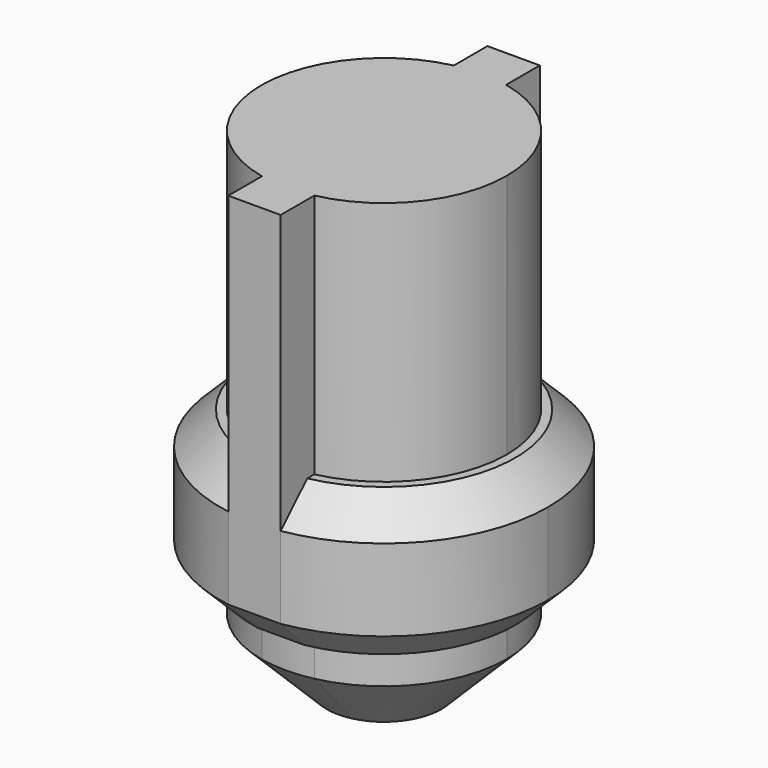
from build123d import *

# Parameters (mm, degrees)
F1_DEPTH     = 7.5
F2_DEPTH     = 7.5
F3_DEPTH     = 4.5
F4_SIZE      = 2
F5_T1_DEPTH  = 6.7433659759
F5_T4_ANGLE  = 220.4864882976
F5_T6_ANGLE  = 220.4864882976
F5_T10_ANGLE = 220.4864882976
F5_T15_ANGLE = 220.4864882976
F5_T20_ANGLE = 220.4864882976
F5_T25_ANGLE = 220.4864882976


# Not quite as in the source:
# - a fillet or chamfer that OpenCascade refuses, or shapes differently, is made with other operations: its cross-section is extruded or revolved along the edge and cut away or added


with BuildPart() as f1:
    # F0 (on Top) → F1 (new body)
    with BuildSketch(Plane.XY):
        with BuildLine():
            ThreePointArc((0.8, -3.6636730203), (2.9208303614, -2.3518609653), (3.75, 0))
            ThreePointArc((3.75, 0), (2.9208303614, 2.3518609653), (0.8, 3.6636730203))
            Line((0.8, 3.6636730203), (0.8, -3.6636730203))
        make_face()
        with BuildLine():
            Line((0.8, -3.6636730203), (0.8, 3.6636730203))
            ThreePointArc((0.8, 3.6636730203), (0, 3.75), (-0.8, 3.6636730203))
            Line((-0.8, 3.6636730203), (-0.8, -3.6636730203))
            ThreePointArc((-0.8, -3.6636730203), (0, -3.75), (0.8, -3.6636730203))
        make_face()
        with BuildLine():
            Line((-0.8, -3.6636730203), (-0.8, 3.6636730203))
            ThreePointArc((-0.8, 3.6636730203), (-3.75, 0), (-0.8, -3.6636730203))
        make_face()
    extrude(amount=-F1_DEPTH)

    # F0 (on Top) → F2 (join)
    with BuildSketch(Plane.XY):
        with BuildLine():
            ThreePointArc((0.8, -3.6636730203), (2.9208303614, -2.3518609653), (3.75, 0))
            ThreePointArc((3.75, 0), (2.9208303614, 2.3518609653), (0.8, 3.6636730203))
            Line((0.8, 3.6636730203), (0.8, -3.6636730203))
        make_face()
        with BuildLine():
            Line((0.8, -3.6636730203), (0.8, 3.6636730203))
            ThreePointArc((0.8, 3.6636730203), (0, 3.75), (-0.8, 3.6636730203))
            Line((-0.8, 3.6636730203), (-0.8, -3.6636730203))
            ThreePointArc((-0.8, -3.6636730203), (0, -3.75), (0.8, -3.6636730203))
        make_face()
        with BuildLine():
            Line((-0.8, -3.6636730203), (-0.8, 3.6636730203))
            ThreePointArc((-0.8, 3.6636730203), (-3.75, 0), (-0.8, -3.6636730203))
        make_face()
        with BuildLine():
            ThreePointArc((-0.8, 3.6636730203), (0, 3.75), (0.8, 3.6636730203))
            Line((0.8, 3.6636730203), (0.8, 4.95))
            Line((0.8, 4.95), (-0.8, 4.95))
            Line((-0.8, 4.95), (-0.8, 3.6636730203))
        make_face()
        with BuildLine():
            Line((0.8, -4.95), (0.8, -3.6636730203))
            ThreePointArc((0.8, -3.6636730203), (0, -3.75), (-0.8, -3.6636730203))
            Line((-0.8, -3.6636730203), (-0.8, -4.95))
            Line((-0.8, -4.95), (0.8, -4.95))
        make_face()
    extrude(amount=F2_DEPTH)

    # F0 (on Top) → F3 (join)
    with BuildSketch(Plane.XY):
        with BuildLine():
            ThreePointArc((0.8, 3.6636730203), (2.9208303614, 2.3518609653), (3.75, 0))
            ThreePointArc((3.75, 0), (2.9208303614, -2.3518609653), (0.8, -3.6636730203))
            Line((0.8, -3.6636730203), (0.8, -4.95))
            ThreePointArc((0.8, -4.95), (3.8179761524, -3.2504704428), (5.0142297514, 0))
            ThreePointArc((5.0142297514, 0), (3.8179761524, 3.2504704428), (0.8, 4.95))
            Line((0.8, 4.95), (0.8, 3.6636730203))
        make_face()
        with BuildLine():
            Line((0.8, -4.95), (0.8, -3.6636730203))
            ThreePointArc((0.8, -3.6636730203), (0, -3.75), (-0.8, -3.6636730203))
            Line((-0.8, -3.6636730203), (-0.8, -4.95))
            Line((-0.8, -4.95), (0.8, -4.95))
        make_face()
        with BuildLine():
            ThreePointArc((-0.8, -3.6636730203), (-3.75, 0), (-0.8, 3.6636730203))
            Line((-0.8, 3.6636730203), (-0.8, 4.95))
            ThreePointArc((-0.8, 4.95), (-5.0142297514, 0), (-0.8, -4.95))
            Line((-0.8, -4.95), (-0.8, -3.6636730203))
        make_face()
        with BuildLine():
            ThreePointArc((-0.8, 3.6636730203), (0, 3.75), (0.8, 3.6636730203))
            Line((0.8, 3.6636730203), (0.8, 4.95))
            Line((0.8, 4.95), (-0.8, 4.95))
            Line((-0.8, 4.95), (-0.8, 3.6636730203))
        make_face()
    extrude(amount=-F3_DEPTH)

    # F4
    f4_edges = [f1.edges().sort_by_distance(p)[0] for p in [
        (0.8, -3.663673, -7.5),
    ]]
    chamfer(f4_edges, length=F4_SIZE)

    # F5: chamfer of 1 on 6 edges, made by hand

    # F5_s2 → F5_t1 (cut)
    with BuildSketch(Plane.YZ.offset(-3.371682988)):
        Polygon((-3.95, -4.5), (-4.95, -3.5), (-4.95, -4.5), align=None)
        Polygon((3.95, -4.5), (4.95, -3.5), (4.95, -4.5), align=None)
    extrude(amount=F5_T1_DEPTH, mode=Mode.SUBTRACT)

    # F5_s3 → F5_t4 (revolve, cut)
    with BuildSketch(Plane(origin=(0, 0, 0), x_dir=(0, 0, 1), z_dir=(0.9382321407, -0.3460064308, 0))):
        Polygon((-4.5, -4.0142297514), (-3.5, -5.0142297514), (-4.5, -5.0142297514), align=None)
    revolve(axis=Axis((0, 0, -4.5), (0, 0, 1)), revolution_arc=F5_T4_ANGLE, mode=Mode.SUBTRACT)

    # F5_s5 → F5_t6 (revolve, cut)
    with BuildSketch(Plane(origin=(0, 0, 0), x_dir=(0, 0, 1), z_dir=(-0.9382321407, 0.3460064308, 0))):
        Polygon((-4.5, -4.0142297514), (-3.5, -5.0142297514), (-4.5, -5.0142297514), align=None)
    revolve(axis=Axis((0, 0, -4.5), (0, 0, 1)), revolution_arc=F5_T6_ANGLE, mode=Mode.SUBTRACT)


with BuildPart() as f5_tool8:
    # F5_s9 → F5_t10 (revolve)
    with BuildSketch(Plane(origin=(0, 0, 0), x_dir=(0, 0, 1), z_dir=(0.9382321407, -0.3460064308, 0))):
        Polygon((-1, -5.0142297514), (0, -4.0142297514), (0, -5.0142297514), align=None)
    revolve(axis=Axis((0, 0, 0), (0, 0, 1)), revolution_arc=F5_T10_ANGLE)

    split(bisect_by=Plane.YZ.offset(0.8), keep=Keep.TOP)


with BuildPart() as f1_1:
    add(f1.part)

    # F5_t7: cut F5_tool8
    add(f5_tool8.part, mode=Mode.SUBTRACT)


with BuildPart() as f5_tool13:
    # F5_s14 → F5_t15 (revolve)
    with BuildSketch(Plane(origin=(0, 0, 0), x_dir=(0, 0, 1), z_dir=(0.9382321407, -0.3460064308, 0))):
        Polygon((-1, -5.0142297514), (0, -4.0142297514), (0, -5.0142297514), align=None)
    revolve(axis=Axis((0, 0, 0), (0, 0, 1)), revolution_arc=F5_T15_ANGLE)

    split(bisect_by=Plane.YZ.offset(-0.8), keep=Keep.BOTTOM)


with BuildPart() as f1_2:
    add(f1_1.part)

    # F5_t12: cut F5_tool13
    add(f5_tool13.part, mode=Mode.SUBTRACT)


with BuildPart() as f5_tool18:
    # F5_s19 → F5_t20 (revolve)
    with BuildSketch(Plane(origin=(0, 0, 0), x_dir=(0, 0, 1), z_dir=(-0.9382321407, 0.3460064308, 0))):
        Polygon((-1, -5.0142297514), (0, -4.0142297514), (0, -5.0142297514), align=None)
    revolve(axis=Axis((0, 0, 0), (0, 0, 1)), revolution_arc=F5_T20_ANGLE)

    split(bisect_by=Plane.YZ.offset(-0.8), keep=Keep.BOTTOM)


with BuildPart() as f1_3:
    add(f1_2.part)

    # F5_t17: cut F5_tool18
    add(f5_tool18.part, mode=Mode.SUBTRACT)


with BuildPart() as f5_tool23:
    # F5_s24 → F5_t25 (revolve)
    with BuildSketch(Plane(origin=(0, 0, 0), x_dir=(0, 0, 1), z_dir=(-0.9382321407, 0.3460064308, 0))):
        Polygon((-1, -5.0142297514), (0, -4.0142297514), (0, -5.0142297514), align=None)
    revolve(axis=Axis((0, 0, 0), (0, 0, 1)), revolution_arc=F5_T25_ANGLE)

    split(bisect_by=Plane.YZ.offset(0.8), keep=Keep.TOP)


with BuildPart() as f1_4:
    add(f1_3.part)

    # F5_t22: cut F5_tool23
    add(f5_tool23.part, mode=Mode.SUBTRACT)


solid = f1_4.part
